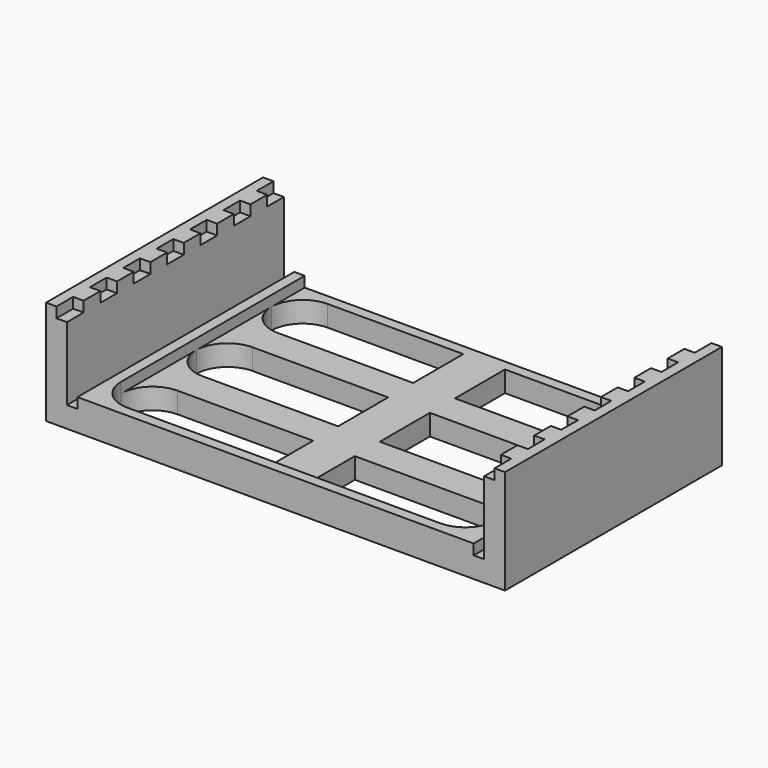
from build123d import *

# Parameters (mm, degrees)
F0_W      = 2200
F0_H      = 1300
F1_DEPTH  = 500
F2_W      = 2000
F2_H      = 400
F3_DEPTH  = 1300
F4_W      = 50
F4_H      = 100
F5_DEPTH  = 50
F6_W      = 50
F6_H      = 100
F7_DEPTH  = 50
F8_W      = 50
F8_H      = 1300
F9_DEPTH  = 50
F10_W     = 1800
F10_H     = 50
F11_DEPTH = 50
F12_W     = 800
F12_H     = 300
F13_DEPTH = 180
F14_R     = 149.99999


# Not quite as in the source:
# - a fillet or chamfer is up to 0.001 mm smaller than in the source, because OpenCascade refuses the exact size


with BuildPart() as f1:
    # F0 (on Top) → F1 (new body)
    with BuildSketch(Plane.XY):
        Rectangle(F0_W, F0_H)
    extrude(amount=-F1_DEPTH)

    # F2 (on face) → F3 (cut)
    with BuildSketch(Plane.XZ.offset(650)):
        with Locations((0, -200)):
            Rectangle(F2_W, F2_H)
    extrude(amount=-F3_DEPTH, mode=Mode.SUBTRACT)

    # F4 (on face) → F5 (cut)
    with BuildSketch(Plane.XY):
        with Locations((-1025, -600)):
            Rectangle(F4_W, F4_H)
        with Locations((-1025, -400)):
            Rectangle(F4_W, F4_H)
        with Locations((-1025, -200)):
            Rectangle(F4_W, F4_H)
        with Locations((-1025, 0)):
            Rectangle(F4_W, F4_H)
        with Locations((-1025, 200)):
            Rectangle(F4_W, F4_H)
        with Locations((-1025, 400)):
            Rectangle(F4_W, F4_H)
        with Locations((-1025, 600)):
            Rectangle(F4_W, F4_H)
    extrude(amount=-F5_DEPTH, mode=Mode.SUBTRACT)

    # F6 (on face) → F7 (cut)
    with BuildSketch(Plane.XY):
        with Locations((1025, 600)):
            Rectangle(F6_W, F6_H)
        with Locations((1025, 400)):
            Rectangle(F6_W, F6_H)
        with Locations((1025, 200)):
            Rectangle(F6_W, F6_H)
        with Locations((1025, 0)):
            Rectangle(F6_W, F6_H)
        with Locations((1025, -200)):
            Rectangle(F6_W, F6_H)
        with Locations((1025, -400)):
            Rectangle(F6_W, F6_H)
        with Locations((1025, -600)):
            Rectangle(F6_W, F6_H)
    extrude(amount=-F7_DEPTH, mode=Mode.SUBTRACT)

    # F8 (on face) → F9 (join)
    with BuildSketch(Plane.XY.offset(-400)):
        with Locations((-925, 0)):
            Rectangle(F8_W, F8_H)
        with Locations((925, 0)):
            Rectangle(F8_W, F8_H)
    extrude(amount=F9_DEPTH)

    # F10 (on face) → F11 (join)
    with BuildSketch(Plane.XY.offset(-400)):
        with Locations((0, -625)):
            Rectangle(F10_W, F10_H)
    extrude(amount=F11_DEPTH)

    # F12 (on face) → F13 (cut)
    with BuildSketch(Plane.XY.offset(-400)):
        with Locations((-500, 450)):
            Rectangle(F12_W, F12_H)
        with Locations((500, 450)):
            Rectangle(F12_W, F12_H)
        with Locations((500, 0)):
            Rectangle(F12_W, F12_H)
        with Locations((-500, 0)):
            Rectangle(F12_W, F12_H)
        with Locations((-500, -450)):
            Rectangle(F12_W, F12_H)
        with Locations((500, -450)):
            Rectangle(F12_W, F12_H)
    extrude(amount=-F13_DEPTH, mode=Mode.SUBTRACT)

    # F14 (radius 150 in the source; OpenCascade refuses exactly that, so slightly less here)
    f14_edges = [f1.edges().sort_by_distance(p)[0] for p in [
        (-900, 600, -450),
        (-900, 300, -450),
        (-900, -150, -450),
        (-900, 150, -450),
        (-900, -600, -425),
        (-900, -300, -450),
        (900, 600, -450),
        (900, 150, -450),
        (900, -300, -450),
        (900, 300, -450),
        (900, -150, -450),
        (900, -600, -425),
    ]]
    fillet(f14_edges, radius=F14_R)


solid = f1.part
